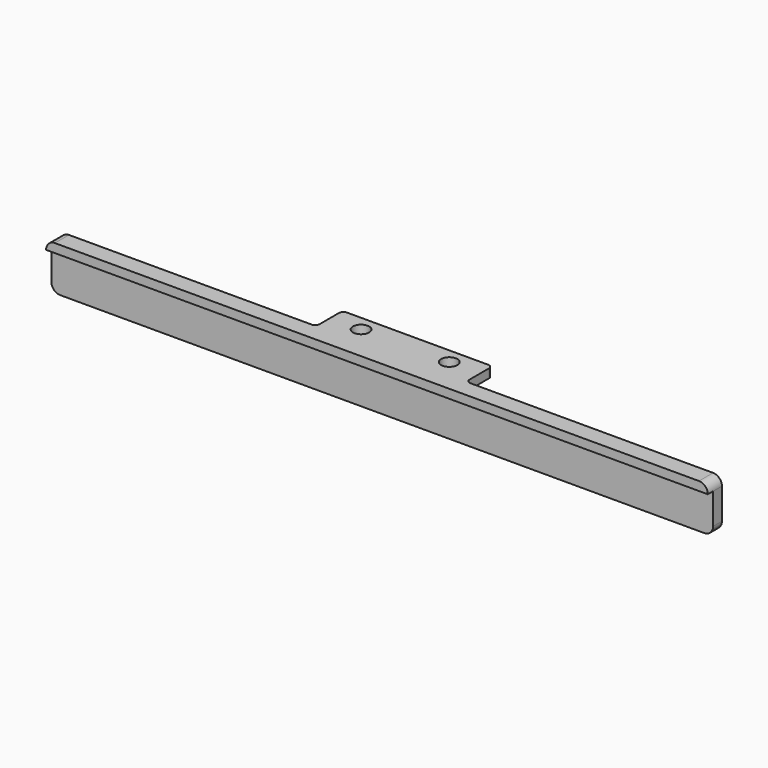
from build123d import *

# Parameters (mm, degrees)
F0_W      = 34
F0_H      = 10
F1_DEPTH  = 11
F2_W      = 2.5
F2_H      = 11
F3_DEPTH  = 58
F4_W      = 2.5
F4_H      = 11
F5_DEPTH  = 58
F6_W      = 7.5
F6_H      = 9
F7_DEPTH  = 92.001
F8_R      = 1.85
F9_DEPTH  = 2.001
F10_R     = 1
F11_W     = 150
F11_H     = 2
F12_DEPTH = 1.5
F13_R     = 1.99999


# Not quite as in the source:
# - a fillet or chamfer is up to 0.001 mm smaller than in the source, because OpenCascade refuses the exact size


with BuildPart() as f1:
    # F0 (on Top) → F1 (new body)
    with BuildSketch(Plane.XY):
        with Locations((-3.2397536635, -4.5336725935)):
            Rectangle(F0_W, F0_H)
    extrude(amount=F1_DEPTH)

    # F2 (on face) → F3 (join)
    with BuildSketch(Plane(origin=(-20.2397536635, 0, 0), x_dir=(0, -1, 0), z_dir=(-1, 0, 0))):
        with Locations((8.2836725935, 5.5)):
            Rectangle(F2_W, F2_H)
    extrude(amount=F3_DEPTH)

    # F4 (on face) → F5 (join)
    with BuildSketch(Plane.YZ.offset(13.7602463365)):
        with Locations((-8.2836725935, 5.5)):
            Rectangle(F4_W, F4_H)
    extrude(amount=F5_DEPTH)

    # F6 (on face) → F7 (cut, through all)
    with BuildSketch(Plane.YZ.offset(13.7602463365)):
        with Locations((-3.2836725935, 4.5)):
            Rectangle(F6_W, F6_H)
    extrude(amount=-F7_DEPTH, mode=Mode.SUBTRACT)

    # F8 (on face) → F9 (cut, through all)
    with BuildSketch(Plane(origin=(0, 0, 9), x_dir=(1, 0, 0), z_dir=(0, 0, -1))):
        with Locations((-13.2397536635, 3.0336725935)):
            Circle(F8_R)
        with Locations((6.7602463365, 3.0336725935)):
            Circle(F8_R)
    extrude(amount=-F9_DEPTH, mode=Mode.SUBTRACT)

    # F10
    f10_edges = [f1.edges().sort_by_distance(p)[0] for p in [
        (-3.239754, -7.033673, 9),
        (-20.239754, -7.033673, 10),
        (13.760246, -7.033673, 10),
        (-20.239754, 0.466327, 10),
        (13.760246, 0.466327, 10),
    ]]
    fillet(f10_edges, radius=F10_R)

    # F11 (on face) → F12 (join)
    with BuildSketch(Plane.XZ.offset(9.5336725935)):
        with Locations((-3.2397536635, 10)):
            Rectangle(F11_W, F11_H)
    extrude(amount=F12_DEPTH)

    # F13 (radius 2 in the source; OpenCascade refuses exactly that, so slightly less here)
    f13_edges = [f1.edges().sort_by_distance(p)[0] for p in [
        (-78.239754, -9.033673, 11),
        (-78.239754, -8.283673, 0),
        (71.760246, -9.033673, 11),
        (71.760246, -8.283673, 0),
    ]]
    fillet(f13_edges, radius=F13_R)


solid = f1.part
